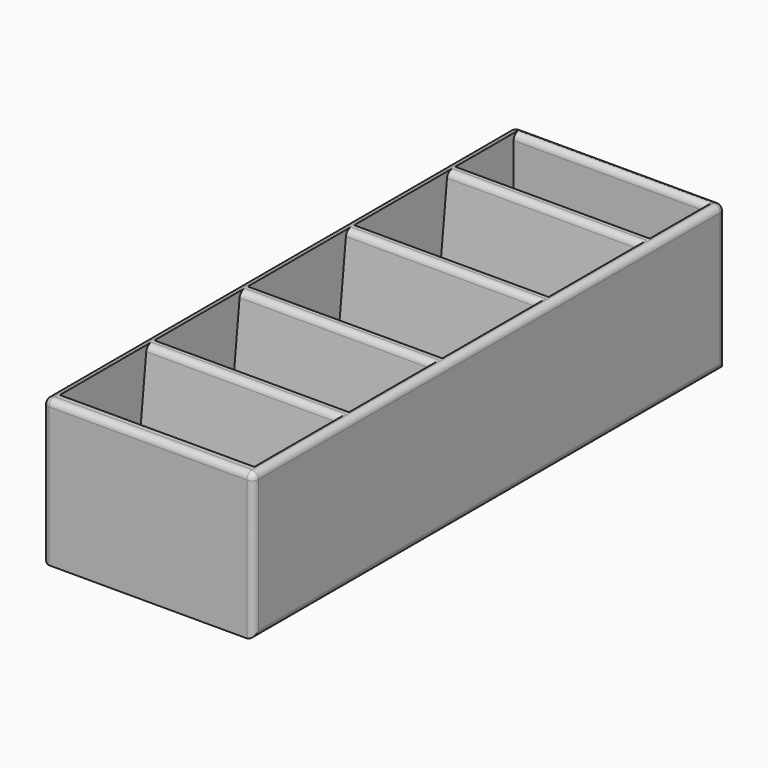
from build123d import *

# Parameters (mm, degrees)
F0_W        = 65
F0_H        = 182
F1_DEPTH    = 45
F2_W        = 60
F2_H        = 175
F3_DEPTH    = 40
F5_DEPTH    = 65
F6_R        = 2
F7_T1_DEPTH = 60


# Not quite as in the source:
# - a fillet or chamfer that OpenCascade refuses, or shapes differently, is made with other operations: its cross-section is extruded or revolved along the edge and cut away or added


with BuildPart() as f1:
    # F0 (on Top) → F1 (new body)
    with BuildSketch(Plane.XY):
        Rectangle(F0_W, F0_H)
    extrude(amount=F1_DEPTH)

    # F2 (on face) → F3 (cut)
    with BuildSketch(Plane.XY.offset(45)):
        Rectangle(F2_W, F2_H)
    extrude(amount=-F3_DEPTH, mode=Mode.SUBTRACT)

    # F4 (on face) → F5 (join)
    with BuildSketch(Plane.YZ.offset(32.5)):
        Polygon((-51, 45), (-54, 45), (-59, 0), (-56, 0), align=None)
        Polygon((-15, 45), (-18, 45), (-23, 0), (-20, 0), align=None)
        Polygon((26, 45), (23, 45), (18, 0), (21, 0), align=None)
        Polygon((65, 45), (62, 45), (57, 0), (65, 0), align=None)
    extrude(amount=-F5_DEPTH)

    # F6
    f6_edges = [f1.edges().sort_by_distance(p)[0] for p in [
        (-32.5, 0, 0),
        (-32.5, 91, 22.5),
        (-32.5, 0, 45),
        (-32.5, -91, 22.5),
        (32.5, 0, 0),
        (32.5, -91, 22.5),
        (32.5, 0, 45),
        (32.5, 91, 22.5),
        (0, -91, 45),
        (0, 91, 45),
    ]]
    fillet(f6_edges, radius=F6_R)

    # F7: fillet of radius 2 on 5 edges, made by hand

    # F7_s2 → F7_t1 (cut)
    with BuildSketch(Plane.YZ.offset(-30)):
        with BuildLine():
            ThreePointArc((-52.2099144137, 45), (-53.5437573385, 44.4902560358), (-54.1976818831, 43.2208630521))
            Line((-54.1976818831, 43.2208630521), (-54, 45))
            Line((-54, 45), (-52.2099144137, 45))
        make_face()
        with BuildLine():
            ThreePointArc((-16.2099144137, 45), (-17.5437573385, 44.4902560358), (-18.1976818831, 43.2208630521))
            Line((-18.1976818831, 43.2208630521), (-18, 45))
            Line((-18, 45), (-16.2099144137, 45))
        make_face()
        with BuildLine():
            ThreePointArc((24.7900855863, 45), (23.4562426615, 44.4902560358), (22.8023181169, 43.2208630521))
            Line((22.8023181169, 43.2208630521), (23, 45))
            Line((23, 45), (24.7900855863, 45))
        make_face()
        with BuildLine():
            ThreePointArc((63.7900855863, 45), (62.4562426615, 44.4902560358), (61.8023181169, 43.2208630521))
            Line((61.8023181169, 43.2208630521), (62, 45))
            Line((62, 45), (63.7900855863, 45))
        make_face()
        with BuildLine():
            ThreePointArc((89.5, 45), (88.0857864376, 44.4142135624), (87.5, 43))
            Line((87.5, 43), (87.5, 45))
            Line((87.5, 45), (89.5, 45))
        make_face()
    extrude(amount=F7_T1_DEPTH, mode=Mode.SUBTRACT)


solid = f1.part
